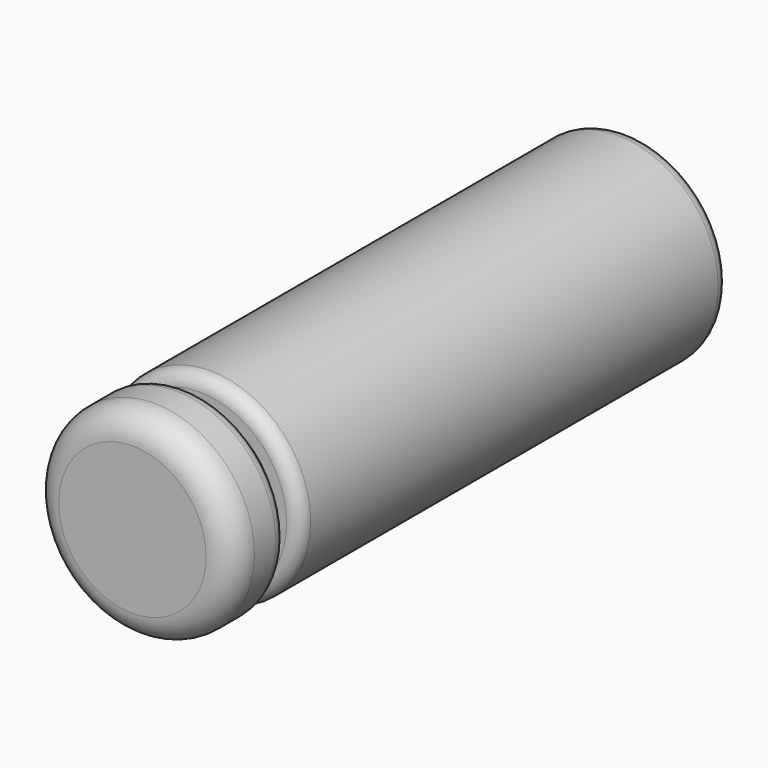
from build123d import *

# Parameters (mm, degrees)
F0_R      = 19.05
F1_DEPTH  = 101.6
F2_R      = 2.54
F5_R      = 14.2875
F5_R_2    = 6.35
F6_DEPTH  = 3.175
F7_R      = 19.05
F7_R_2    = 14.2875
F8_DEPTH  = 25.4
F10_R     = 19.05
F11_DEPTH = 12.7
F12_R     = 2.54
F13_R     = 5.08
F3_R      = 6.35
F14_DEPTH = 104.775


# Not quite as in the source:
# - a feature names something its author has since deleted; it is built from what else it names


with BuildPart() as f1:
    # F0 (on Front) → F1 (new body)
    with BuildSketch(Plane.XZ):
        Circle(F0_R)
    extrude(amount=F1_DEPTH)

    # F2
    f2_edges = [f1.edges().sort_by_distance(p)[0] for p in [
        (-19.05, -101.6, 0),
        (-19.05, 0, 0),
    ]]
    fillet(f2_edges, radius=F2_R)

    # F5 (on face) → F6 (join)
    with BuildSketch(Plane.XZ.offset(101.6)):
        Circle(F5_R)
        Circle(F5_R_2, mode=Mode.SUBTRACT)
    extrude(amount=F6_DEPTH)

    # F10 (on face) → F11 (join)
    with BuildSketch(Plane.XZ.offset(104.775)):
        Circle(F10_R)
    extrude(amount=F11_DEPTH)

    # F12
    f12_edges = [f1.edges().sort_by_distance(p)[0] for p in [
        (-19.05, -104.775, 0),
    ]]
    fillet(f12_edges, radius=F12_R)

    # F13
    f13_edges = [f1.edges().sort_by_distance(p)[0] for p in [
        (-19.05, -117.475, 0),
    ]]
    fillet(f13_edges, radius=F13_R)

    # F3 (on face) → F14 (cut, through all)
    with BuildSketch(Plane(origin=(0, 0, 0), x_dir=(-1, 0, 0), z_dir=(0, 1, 0))):
        Circle(F3_R)
    extrude(amount=-F14_DEPTH, mode=Mode.SUBTRACT)


with BuildPart() as f8:
    # F7 (on face) → F8 (new body)
    with BuildSketch(Plane.XZ.offset(104.775)):
        Circle(F7_R)
        Circle(F7_R_2, mode=Mode.SUBTRACT)
    extrude(amount=F8_DEPTH)


solid = f1.part
